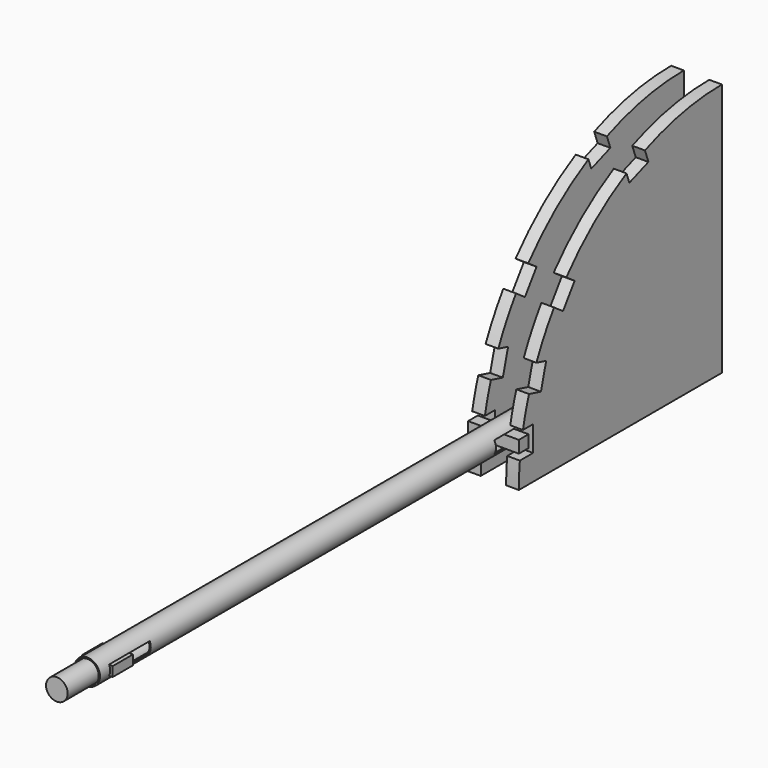
from build123d import *

# Parameters (mm, degrees)
F2_DEPTH       = 5
F5_R           = 5
F5_R_2         = 4.5
F6_DEPTH       = 300
F7_W           = 20
F7_H           = 4
F8_DEPTH       = 25
F9_R           = 4.25
F10_DEPTH      = 15
F10_DEPTH_BACK = 15
F11_W          = 10
F11_H          = 3.8
F12_DEPTH      = 6
F12_DEPTH_BACK = 6
F13_W          = 10
F13_H          = 5
F14_DEPTH      = 25
F14_DEPTH_BACK = 25
F15_W          = 4.8
F15_H          = 4.8
F16_DEPTH      = 10
F16_DEPTH_BACK = 10
F17_D          = 5
F17_DEPTH      = 15.001
F17_2_D        = 5
F17_2_DEPTH    = 15.001


with BuildPart() as f2:
    # F1 (on offset) → F2 (new body)
    with BuildSketch(Plane.YZ.offset(5)):
        with BuildLine():
            ThreePointArc((-84.4987437107, -5), (-84.874607311, -9.993722494), (-85, -15))
            Line((-85, -15), (15, -15))
            Line((15, -15), (15, 85))
            ThreePointArc((15, 85), (-4.3142117375, 83.1170791705), (-22.9010808434, 77.5392244991))
            Line((-22.9010808434, 77.5392244991), (-21.1909801268, 72.8407613952))
            Line((-21.1909801268, 72.8407613952), (-30.5879063346, 69.420559962))
            Line((-30.5879063346, 69.420559962), (-31.9897514765, 73.2720978349))
            ThreePointArc((-31.9897514765, 73.2720978349), (-47.9632403067, 62.6893195367), (-61.625049246, 49.2541969684))
            Line((-61.625049246, 49.2541969684), (-57.5292890245, 46.3863147866))
            Line((-57.5292890245, 46.3863147866), (-63.265053388, 38.1947943437))
            Line((-63.265053388, 38.1947943437), (-67.6631433607, 41.2743700963))
            ThreePointArc((-67.6631433607, 41.2743700963), (-72.3668719499, 33.6521293028), (-76.3697118886, 25.6395835288))
            Line((-76.3697118886, 25.6395835288), (-71.5400827572, 24.3454883033))
            Line((-71.5400827572, 24.3454883033), (-74.1282732082, 14.6862300404))
            Line((-74.1282732082, 14.6862300404), (-79.9895533557, 16.2567553225))
            ThreePointArc((-79.9895533557, 16.2567553225), (-81.6485963638, 10.6719461845), (-82.9795897113, 5))
            Line((-82.9795897113, 5), (-77.9795897113, 5))
            Line((-77.9795897113, 5), (-77.9795897113, -5))
            Line((-77.9795897113, -5), (-84.4987437107, -5))
        make_face()
    extrude(amount=F2_DEPTH)


with BuildPart() as f3_1:
    # F3: instance of F2
    add(f2.part.mirror(Plane.YZ))

    # F17 (through all, one way)
    with BuildSketch(Plane.YZ.offset(5)):
        with Locations((0, 0)):
            Circle(F17_D / 2)
    extrude(amount=-F17_DEPTH, mode=Mode.SUBTRACT)


with BuildPart() as f6:
    # F5 (on offset) → F6 (new body)
    with BuildSketch(Plane.XZ.offset(-15)):
        Circle(F5_R)
        Circle(F5_R_2, mode=Mode.SUBTRACT)
    extrude(amount=F6_DEPTH)

    # F7 (on offset) → F8 (cut)
    with BuildSketch(Plane.YZ.offset(5)):
        with Locations((-270, 0)):
            Rectangle(F7_W, F7_H)
    extrude(amount=-F8_DEPTH, mode=Mode.SUBTRACT)



with BuildPart() as f10:
    # F9 (on face) → F10 (new body, two sides)
    with BuildSketch(Plane.XZ.offset(285)) as f10_sk:
        Circle(F9_R)
    extrude(amount=F10_DEPTH)
    extrude(f10_sk.sketch, amount=-F10_DEPTH_BACK)


with BuildPart() as f6_1:
    add(f6.part)

    add(f10.part)  # F12 merges F10
    # F11 (on Right) → F12 (join, two sides)
    with BuildSketch(Plane.YZ) as f12_sk:
        with Locations((-275, 0)):
            Rectangle(F11_W, F11_H)
    extrude(amount=F12_DEPTH)
    extrude(f12_sk.sketch, amount=-F12_DEPTH_BACK)

    # F13 (on Right) → F14 (cut, two sides)
    with BuildSketch(Plane.YZ) as f14_sk:
        with Locations((-85, 0)):
            Rectangle(F13_W, F13_H)
    extrude(amount=F14_DEPTH, mode=Mode.SUBTRACT)
    extrude(f14_sk.sketch, amount=-F14_DEPTH_BACK, mode=Mode.SUBTRACT)

    # F17#2 (through all, one way)
    with BuildSketch(Plane.YZ.offset(5)):
        with Locations((0, 0)):
            Circle(F17_2_D / 2)
    extrude(amount=-F17_2_DEPTH, mode=Mode.SUBTRACT)


with BuildPart() as f16:
    # F15 (on Right) → F16 (new body, two sides)
    with BuildSketch(Plane.YZ) as f16_sk:
        with Locations((-82.6, 0)):
            Rectangle(F15_W, F15_H)
    extrude(amount=F16_DEPTH)
    extrude(f16_sk.sketch, amount=-F16_DEPTH_BACK)


solid = Compound([f2.part, f3_1.part, f6_1.part, f16.part])
